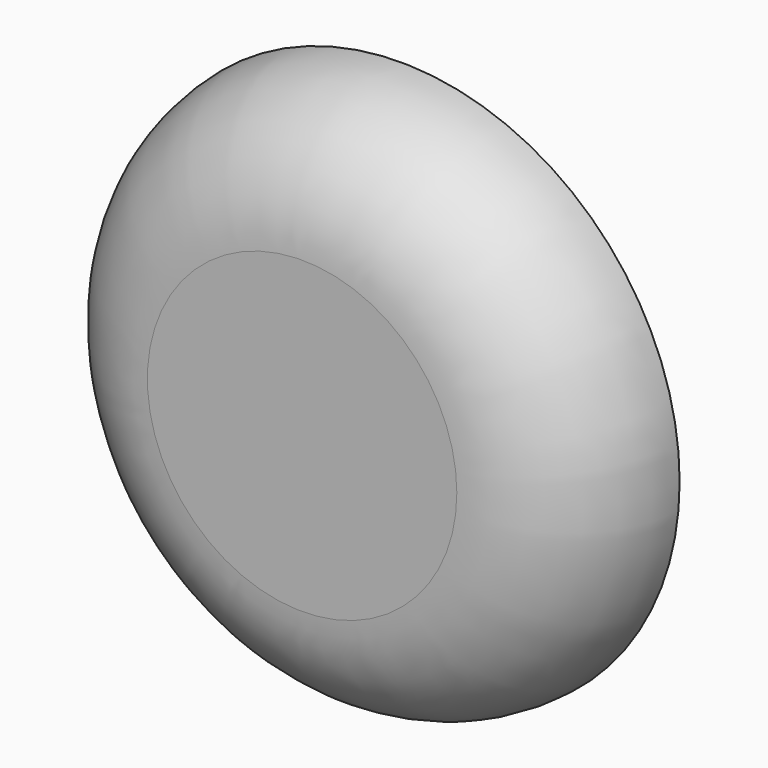
from build123d import *

# Parameters (mm, degrees)
F0_R     = 4.5
F1_DEPTH = 2
F2_R     = 1.99999
F3_R     = 1.35
F4_DEPTH = 3


# Not quite as in the source:
# - a fillet or chamfer is up to 0.001 mm smaller than in the source, because OpenCascade refuses the exact size


with BuildPart() as f1:
    # F0 (on Front) → F1 (new body)
    with BuildSketch(Plane.XZ):
        Circle(F0_R)
    extrude(amount=F1_DEPTH)

    # F2 (radius 2 in the source; OpenCascade refuses exactly that, so slightly less here)
    f2_edges = [f1.edges().sort_by_distance(p)[0] for p in [
        (-4.5, -2, 0),
    ]]
    fillet(f2_edges, radius=F2_R)

    # F3 (on face) → F4 (join)
    with BuildSketch(Plane(origin=(0, 0, 0), x_dir=(-1, 0, 0), z_dir=(0, 1, 0))):
        Circle(F3_R)
    extrude(amount=F4_DEPTH)


solid = f1.part
